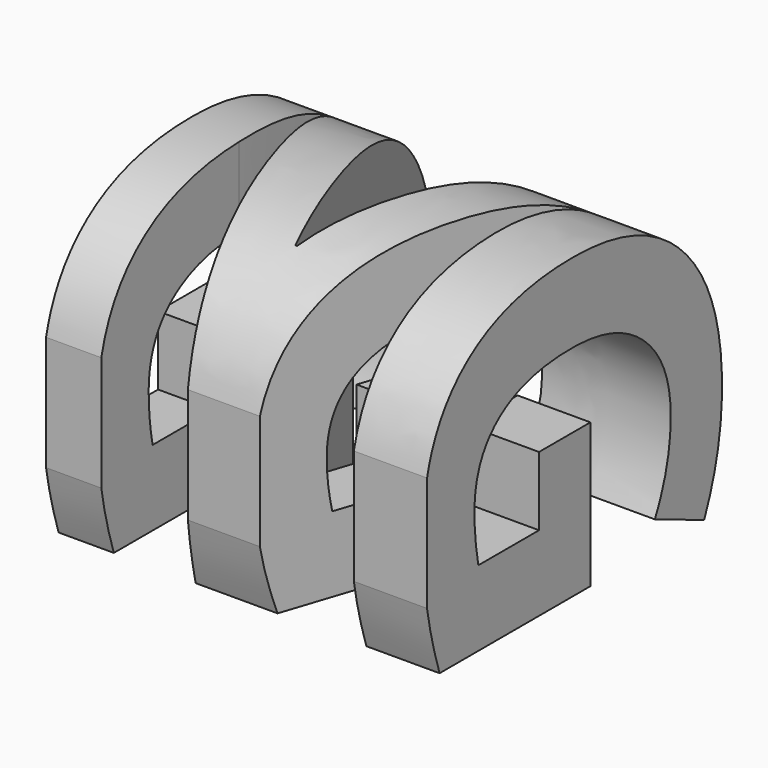
from build123d import *

# Parameters (mm, degrees)
F0_TEXT_SIZE = 108.9547156963
F1_DEPTH     = 100
F2_TEXT_SIZE = 106.9444444444
F1_FACE1_W   = 77.7834525026
F1_FACE1_H   = 100
F3_DEPTH     = 80


# Not quite as in the source:
# - Text() gives the source's letters only with a copy of the font that has no kerning and outlines rounded to 1/6400 em; it was checked with that copy


with BuildPart() as f1:
    # F0 (on Top) → F1 (new body)
    with BuildSketch(Plane.XY):
        with Locations((0, 0)):
            Text('M', F0_TEXT_SIZE, font='Open Sans', font_style=FontStyle.BOLD, text_align=(TextAlign.LEFT, TextAlign.BOTTOM))
    extrude(amount=F1_DEPTH)

    # F2 (on face) + F1_face1 (on face) → F3 (intersect)
    with BuildSketch(Plane.YZ.offset(92.9349676541)):
        with Locations(Location((0, 96.25), (0, 0, -90))):
            Text('G', F2_TEXT_SIZE, font='Open Sans', font_style=FontStyle.BOLD, text_align=(TextAlign.LEFT, TextAlign.BOTTOM))
    with BuildSketch(Plane(origin=(9.7889002383, 38.8917262513, 50), x_dir=(0, -1, 0), z_dir=(-1, 0, 0))):
        Rectangle(F1_FACE1_W, F1_FACE1_H)
    extrude(amount=-F3_DEPTH, dir=(1, 0, 0), mode=Mode.INTERSECT)


solid = f1.part
